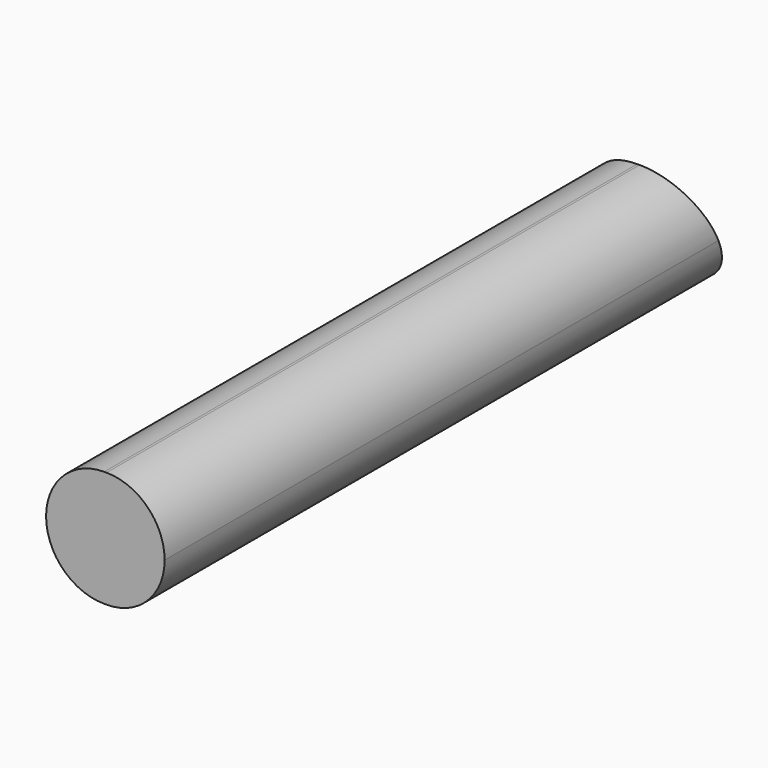
from build123d import *

# Parameters (mm, degrees)
F2_DEPTH = 12.954
F3_R     = 6.34999


# Not quite as in the source:
# - a fillet or chamfer is up to 0.001 mm smaller than in the source, because OpenCascade refuses the exact size


with BuildPart() as f2:
    # F1 (on Right) → F2 (new body)
    with BuildSketch(Plane.YZ):
        Polygon((-39.228890075, 12.7), (-39.228890075, 0), (39.228890075, 0), (33.5844452765, 12.7), align=None)
    extrude(amount=F2_DEPTH)

    # F3 (radius 6.35 in the source; OpenCascade refuses exactly that, so slightly less here)
    f3_edges = [f2.edges().sort_by_distance(p)[0] for p in [
        (12.954, 0, 0),
        (12.954, -2.822222, 12.7),
        (0, -2.822222, 12.7),
        (0, 0, 0),
    ]]
    fillet(f3_edges, radius=F3_R)


solid = f2.part
